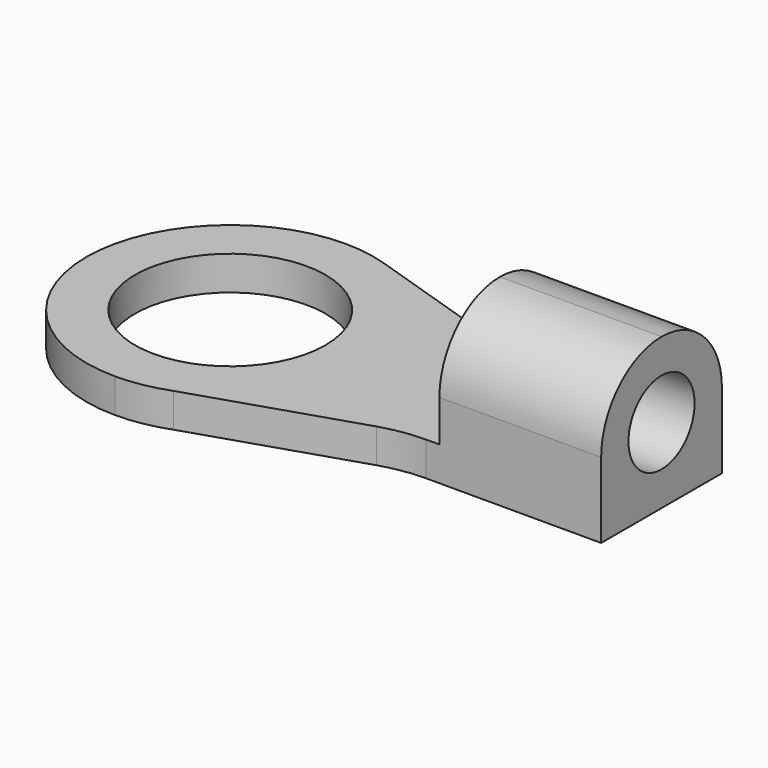
from build123d import *

# Parameters (mm, degrees)
F0_R     = 2.65
F1_DEPTH = 0.95
F2_W     = 4.5
F2_H     = 4.2
F3_DEPTH = 3.25
F4_R     = 2.09999
F5_R     = 1.15
F6_DEPTH = 25


# Not quite as in the source:
# - a fillet or chamfer is up to 0.001 mm smaller than in the source, because OpenCascade refuses the exact size


with BuildPart() as f1:
    # F0 (on Top) → F1 (new body)
    with BuildSketch(Plane.XY):
        with BuildLine():
            Line((11.1295213641, 1.9), (16, 1.9))
            Line((16, 1.9), (16, 6.1))
            Line((16, 6.1), (11.1313788328, 6.1))
            ThreePointArc((11.1313788328, 6.1), (10.5077213988, 6.1489176919), (9.8993179059, 6.2944742975))
            Line((9.8993179059, 6.2944742975), (5.2320609269, 7.8055257025))
            ThreePointArc((5.2320609269, 7.8055257025), (4.623657434, 7.9510823081), (4, 8))
            ThreePointArc((4, 8), (1.1715728753, 6.8284271247), (0, 4))
            ThreePointArc((0, 4), (1.1715728753, 1.1715728753), (4, 0))
            ThreePointArc((4, 0), (4.7206487948, 0.0654523367), (5.4177135157, 0.2596673427))
            Line((5.4177135157, 0.2596673427), (9.9009095946, 1.7066406607))
            ThreePointArc((9.9009095946, 1.7066406607), (10.5076542734, 1.8513644886), (11.1295213641, 1.9))
        make_face()
        with Locations((4, 4)):
            Circle(F0_R, mode=Mode.SUBTRACT)
    extrude(amount=F1_DEPTH)

    # F2 (on face) → F3 (join)
    with BuildSketch(Plane.XY.offset(0.95)):
        with Locations((13.75, 4)):
            Rectangle(F2_W, F2_H)
    extrude(amount=F3_DEPTH)

    # F4 (radius 2.1 in the source; OpenCascade refuses exactly that, so slightly less here)
    f4_edges = [f1.edges().sort_by_distance(p)[0] for p in [
        (13.75, 6.1, 4.2),
        (13.75, 1.9, 4.2),
    ]]
    fillet(f4_edges, radius=F4_R)

    # F5 (on face) → F6 (cut)
    with BuildSketch(Plane.YZ.offset(16)):
        with Locations((4, 2.1)):
            Circle(F5_R)
    extrude(amount=-F6_DEPTH, mode=Mode.SUBTRACT)


solid = f1.part
